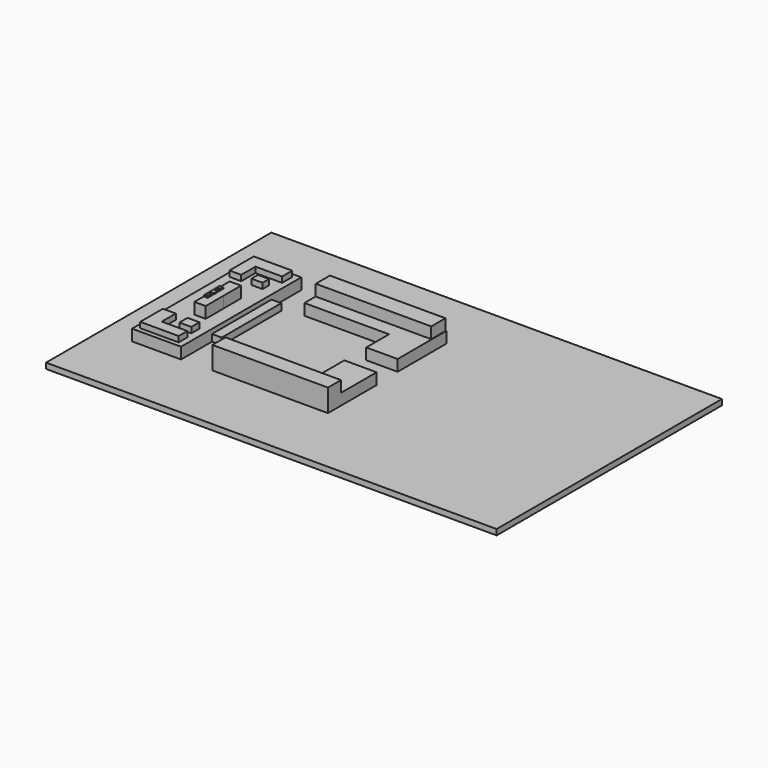
from build123d import *

# Parameters (mm, degrees)
F0_W      = 1016
F0_H      = 635
F1_DEPTH  = 12.7
F2_W      = 190.9023970366
F2_H      = 72.670340538
F2_W_2    = 110.4675829411
F2_H_2    = 338.8325423002
F2_W_3    = 187.6850500703
F2_H_3    = 73.4205134213
F3_DEPTH  = 25.4
F4_W      = 260.4392468929
F4_H      = 36.7102567106
F4_H_2    = 39.9852208793
F4_W_2    = 25.2980589867
F4_H_3    = 0.1311842352
F5_DEPTH  = 25.4
F6_W      = 29.0026068687
F6_H      = 39.524897933
F6_W_2    = 26.9005596638
F6_H_2    = 22.802144289
F6_W_3    = 26.5395641327
F6_H_3    = 40.0708019733
F6_W_4    = 25.1247286797
F6_H_4    = 17.9900527
F7_DEPTH  = 12.7
F8_W      = 8.947044611
F8_H      = 11.3622983918
F8_W_2    = 8.928835392
F8_H_2    = 11.6621851921
F8_W_3    = 8.7315738201
F8_H_3    = 12.1389040723
F9_DEPTH  = 2.54
F10_R     = 4.1746501932
F10_R_2   = 4.2690475455
F11_DEPTH = 0.762
F12_R     = 0.76199
F13_W     = 21.8863785267
F13_H     = 167.8882390261
F14_DEPTH = 15.24


# Not quite as in the source:
# - a fillet or chamfer is up to 0.001 mm smaller than in the source, because OpenCascade refuses the exact size


with BuildPart() as f1:
    # F0 (on Top) → F1 (new body)
    with BuildSketch(Plane.XY):
        Rectangle(F0_W, F0_H)
    extrude(amount=-F1_DEPTH)

    # F2 (on face) → F3 (join)
    with BuildSketch(Plane.XY):
        Polygon((-73.4143704176, 178.6967664957), (-73.4143704176, 106.0264259577), (-73.4143704176, 41.7220070958), (-2.6750040706, 41.7220070958), (-2.6750040706, 178.8768768311), (-73.4143704176, 178.8768768311), align=None)
        with Locations((-168.8655689359, 142.3615962267)):
            Rectangle(F2_W, F2_H)
        with Locations((-385.0155323744, 9.5723941922)):
            Rectangle(F2_W_2, F2_H_2)
        with Locations((-166.5967218578, -121.2908085436)):
            Rectangle(F2_W_3, F2_H_3)
        Polygon((-72.7541968226, -84.5805518329), (-72.7541968226, -158.0010652542), (0, -158.0010652542), (0, -20.846195519), (-72.7541968226, -20.846195519), align=None)
    extrude(amount=F3_DEPTH)

    # F4 (on face) → F5 (join)
    with BuildSketch(Plane.XY.offset(25.4)):
        with Locations((-130.2196234465, -139.6459368989)):
            Rectangle(F4_W, F4_H)
        with Locations((-133.8504105806, 157.6813366264)):
            Rectangle(F4_W, F4_H_2)
        Polygon((-362.4670803547, 0.1311842352), (-362.4670803547, 0), (-387.7651393414, 0), (-387.7651393414, -49.7534926981), (-362.2698187828, -49.7534926981), (-362.2698187828, 0.1311842352), align=None)
        with Locations((-375.116109848, 0.0655921176)):
            Rectangle(F4_W_2, F4_H_3)
        Polygon((-387.9624009132, 0), (-387.7651393414, 0), (-387.7651393414, 0.1311842352), (-362.4670803547, 0.1311842352), (-362.4670803547, 49.8846769333), (-387.9624009132, 49.8846769333), align=None)
    extrude(amount=F5_DEPTH)

    # F6 (on face) → F7 (join)
    with BuildSketch(Plane.XY.offset(25.4)):
        Polygon((-343.3714807034, -149.6838778257), (-343.3714807034, -125.3397166729), (-400.9214937687, -125.3397166729), (-429.9241006374, -125.3397166729), (-429.9241006374, -149.6838778257), align=None)
        with Locations((-415.4227972031, -105.5772677064)):
            Rectangle(F6_W, F6_H)
        with Locations((-360.9930127859, -97.2158908844)):
            Rectangle(F6_W_2, F6_H_2)
        Polygon((-342.8669273853, 141.4012908936), (-342.8669273853, 169.8563098907), (-429.579526186, 169.8563098907), (-429.579526186, 141.4012908936), (-403.0399620533, 141.4012908936), align=None)
        with Locations((-416.3097441196, 121.3658899069)):
            Rectangle(F6_W_3, F6_H_3)
        with Locations((-367.4284219742, 110.3255152702)):
            Rectangle(F6_W_4, F6_H_4)
    extrude(amount=F7_DEPTH)

    # F8 (on face) → F9 (join)
    with BuildSketch(Plane.XY.offset(50.8)):
        with Locations((-383.2916170359, -1.178430859)):
            Rectangle(F8_W, F8_H)
        with Locations((-383.4979832172, 15.6762860715)):
            Rectangle(F8_W_2, F8_H_2)
        with Locations((-383.3993524313, -16.8637591414)):
            Rectangle(F8_W_3, F8_H_3)
    extrude(amount=F9_DEPTH)

    # F10 (on face) → F11 (join)
    with BuildSketch(Plane.XY.offset(53.34)):
        with Locations((-383.3409547806, -17.0078240335)):
            Circle(F10_R)
        with Locations((-383.3993524313, 15.7660990953)):
            Circle(F10_R_2)
    extrude(amount=F11_DEPTH)

    # F12 (radius 0.762 in the source; OpenCascade refuses exactly that, so slightly less here)
    f12_edges = [f1.edges().sort_by_distance(p)[0] for p in [
        (-387.515605, -17.007824, 54.102),
        (-387.6684, 15.766099, 54.102),
    ]]
    fillet(f12_edges, radius=F12_R)

    # F13 (on face) → F14 (join)
    with BuildSketch(Plane.XY):
        with Locations((-318.8385516405, 11.3731846213)):
            Rectangle(F13_W, F13_H)
    extrude(amount=F14_DEPTH)


solid = f1.part
